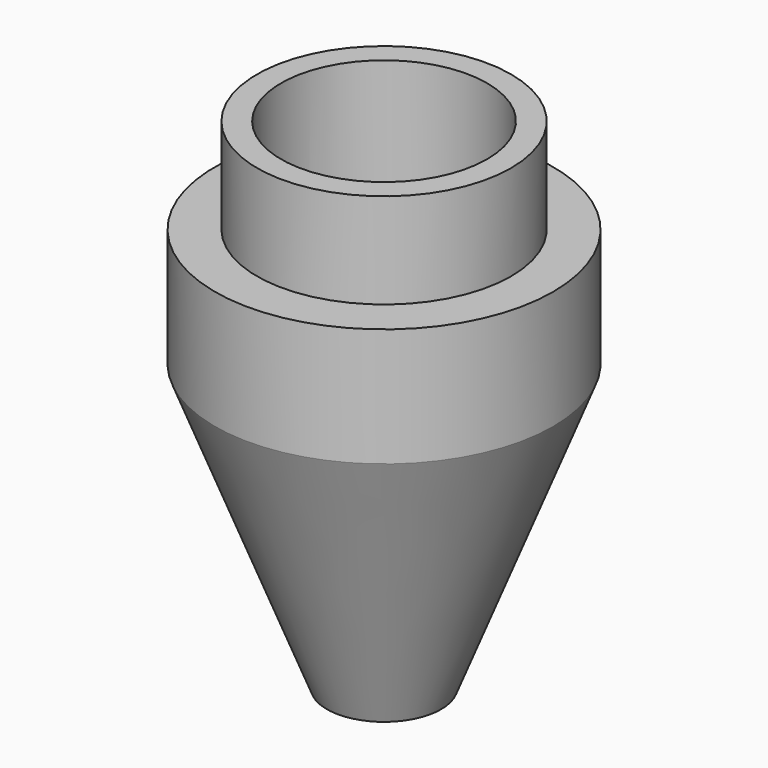
from build123d import *

# Parameters (mm, degrees)
F0_R      = 9.335
F1_DEPTH  = 7
F2_R      = 12.425
F2_R_2    = 9.335
F3_DEPTH  = 8.7
F3_FACE_R = 12.425
F5_R      = 4.2
F8_R      = 7.57
F10_DEPTH = 15.7
F11_R     = 7.57
F9_R      = 2.1
F13_R     = 2.15
F14_REACH = 30.9321184182


with BuildPart() as f1:
    # F0 (on Top) → F1 (new body)
    with BuildSketch(Plane.XY):
        Circle(F0_R)
    extrude(amount=-F1_DEPTH)

    # F2 (on face) → F3 (join)
    with BuildSketch(Plane(origin=(0, 0, -7), x_dir=(1, 0, 0), z_dir=(0, 0, -1))):
        Circle(F2_R)
        Circle(F2_R_2, mode=Mode.SUBTRACT)
        Circle(F2_R_2)
    extrude(amount=F3_DEPTH)

    # F3_face (on face) → F6 section 0
    with BuildSketch(Plane(origin=(0, 0, -15.7), x_dir=(1, 0, 0), z_dir=(0, 0, -1))):
        Circle(F3_FACE_R)
    # F5 (on offset) → F6 section 1
    with BuildSketch(Plane(origin=(0, 0, -36.675), x_dir=(1, 0, 0), z_dir=(0, 0, -1))):
        Circle(F5_R)
    loft()

    # F8 (on face) → F10 (cut)
    with BuildSketch(Plane.XY):
        Circle(F8_R)
    extrude(amount=-F10_DEPTH, mode=Mode.SUBTRACT)

    # F11 (on face) → F12 section 0
    with BuildSketch(Plane.XY.offset(-15.7)):
        Circle(F11_R)
    # F9 (on face) → F12 section 1
    with BuildSketch(Plane(origin=(0, 0, -36.675), x_dir=(1, 0, 0), z_dir=(0, 0, -1))):
        Circle(F9_R)
    loft(mode=Mode.SUBTRACT)

    f14_end = f1.faces().sort_by_distance((-7.57, 0, -7.85))[0]
    # F13 (on offset) → F14 (cut, up to a face of the model that its end follows)
    with BuildSketch(Plane.YZ.offset(-12.425)):
        with Locations((0, -11.35)):
            Circle(F13_R)
    f14_long = extrude(amount=F14_REACH, mode=Mode.PRIVATE)
    add(split(f14_long, bisect_by=f14_end, keep=Keep.ALL, mode=Mode.PRIVATE).solids().sort_by_distance((-12.425, 0, -11.35))[0], mode=Mode.SUBTRACT)


solid = f1.part
